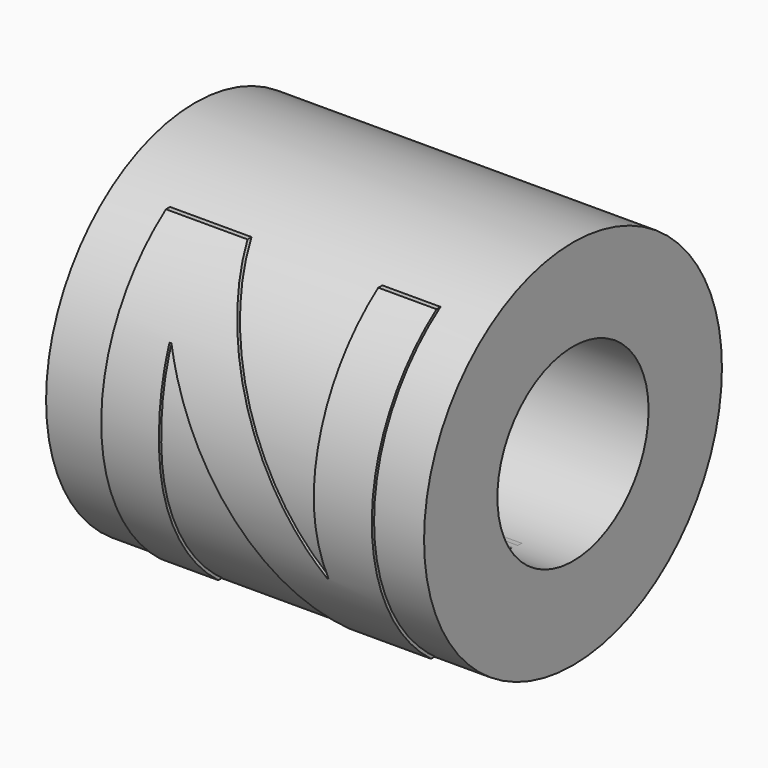
from build123d import *

# Parameters (mm, degrees)
F0_R         = 1
F0_R_2       = 0.985
F0_R_3       = 0.5
F1_DEPTH     = 2
F2_TEXT_SIZE = 2.2604994431
F3_REACH     = 3.1582171497
F4_DEPTH     = 2


# Not quite as in the source:
# - Text() gives the source's letters only with a copy of the font that has no kerning and outlines rounded to 1/6400 em; it was checked with that copy


with BuildPart() as f1:
    # F0 (on Right) → F1 (new body)
    with BuildSketch(Plane.YZ):
        Circle(F0_R)
        Circle(F0_R_2, mode=Mode.SUBTRACT)
        Circle(F0_R_2)
        Circle(F0_R_3, mode=Mode.SUBTRACT)
    extrude(amount=F1_DEPTH)

    f3_end = f1.faces().sort_by_distance((1, -1, 0))[0]
    # F2 (on Front) → F3 (intersect, up to a face of the model that its end follows)
    with BuildSketch(Plane.XZ):
        with Locations((0.1008149993, -0.7936101756)):
            Text('N', F2_TEXT_SIZE, font='Open Sans', font_style=FontStyle.BOLD, text_align=(TextAlign.LEFT, TextAlign.BOTTOM))
    f3_long = extrude(amount=F3_REACH, mode=Mode.PRIVATE)
    add(split(f3_long, bisect_by=f3_end, keep=Keep.BOTTOM, mode=Mode.PRIVATE), mode=Mode.INTERSECT)


with BuildPart() as f4:
    # F0 (on Right) → F4 (new body)
    with BuildSketch(Plane.YZ):
        Circle(F0_R_2)
        Circle(F0_R_3, mode=Mode.SUBTRACT)
    extrude(amount=F4_DEPTH)


solid = Compound([f1.part, f4.part])
